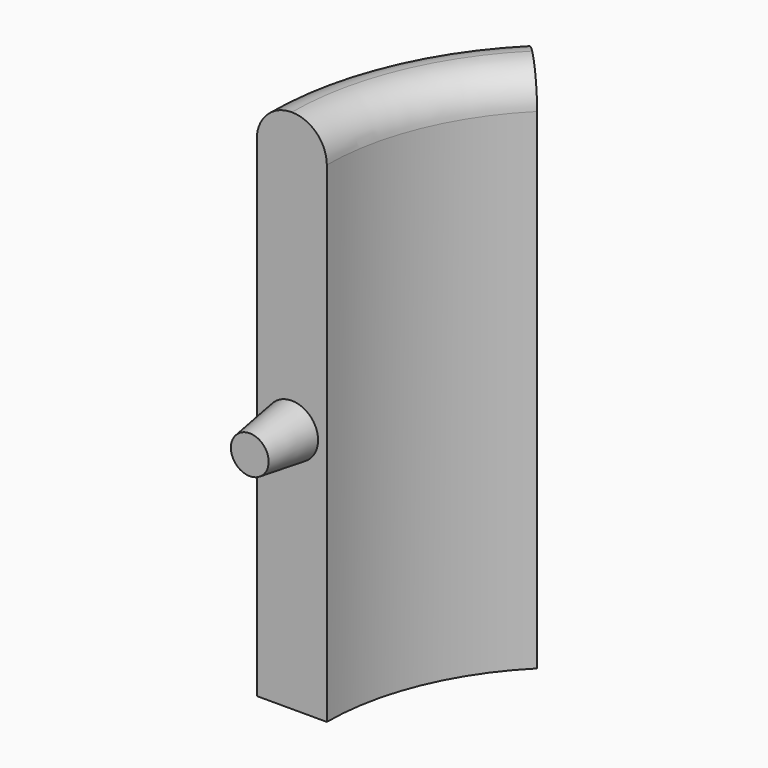
from build123d import *

# Parameters (mm, degrees)
F0_W     = 89.9249566834
F0_H     = 150
F1_ANGLE = 45
F2_T     = -20
F3_R     = 7.5
F4_DEPTH = 15
F4_TAPER = 8
F5_R     = 7.5
F6_DEPTH = 15
F6_TAPER = 8
F7_R     = 9.99999


# Not quite as in the source:
# - a fillet or chamfer is up to 0.001 mm smaller than in the source, because OpenCascade refuses the exact size
# - a feature names something its author has since deleted; it is built from what else it names


with BuildPart() as f1:
    # F0 (on Front) → F1 (revolve)
    with BuildSketch(Plane.XZ):
        with Locations((82.3541893682, 224.1176688539)):
            Rectangle(F0_W, F0_H)
    revolve(axis=Axis((127.3166677099, 0, 224.1176688539), (0, 0, -1)), revolution_arc=F1_ANGLE)

    # F2
    f2_openings = [f1.faces().sort_by_distance(p)[0] for p in [
        (82.354189, 0, 224.117669),
        (95.523394, 31.793273, 224.117669),
        (73.342731, 22.356737, 149.117669),
        (73.342731, 22.356737, 299.117669),
    ]]
    offset(amount=F2_T, openings=f2_openings)

    # F3 (on face) → F4 (join)
    with BuildSketch(Plane.XZ):
        with Locations((47.3917110264, 219.1176688539)):
            Circle(F3_R)
    extrude(amount=F4_DEPTH, taper=F4_TAPER)

    # F5 (on face) → F6 (cut)
    with BuildSketch(Plane(origin=(63.6583338549, 63.6583338549, 0), x_dir=(-0.7071067812, 0.7071067812, 0), z_dir=(0.7071067812, 0.7071067812, 0))):
        with Locations((-9.8187575006, 219.1176688539)):
            Circle(F5_R)
    extrude(amount=-F6_DEPTH, taper=F6_TAPER, mode=Mode.SUBTRACT)

    # F7 (radius 10 in the source; OpenCascade refuses exactly that, so slightly less here)
    f7_edges = [f1.edges().sort_by_distance(p)[0] for p in [
        (44.236841, 34.412791, 299.117669),
        (62.714431, 26.759122, 299.117669),
    ]]
    fillet(f7_edges, radius=F7_R)


solid = f1.part
